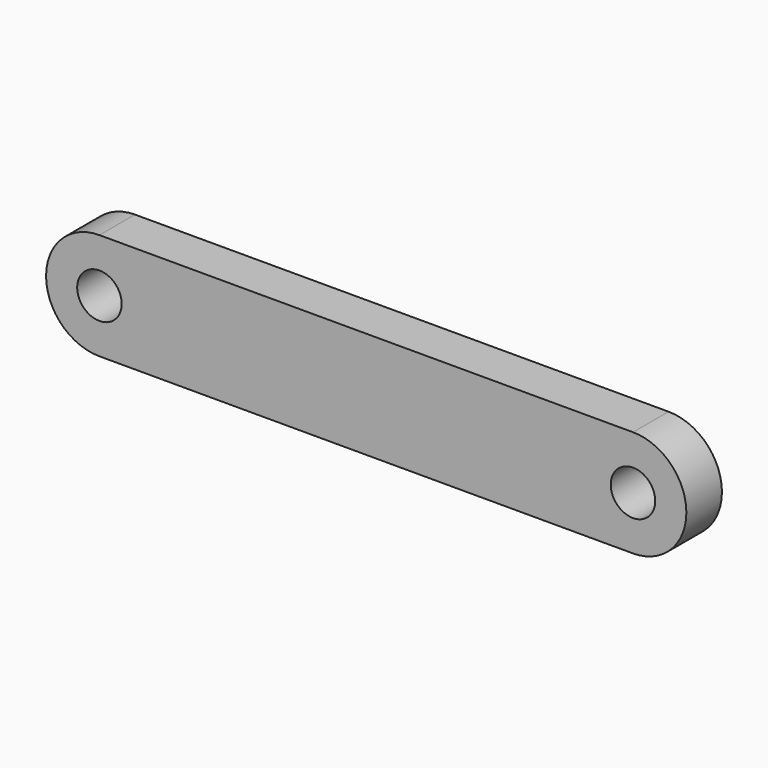
from build123d import *

# Parameters (mm, degrees)
F0_R     = 2.5
F1_DEPTH = 5


# Not quite as in the source:
# - a feature names something its author has since deleted; it is built from what else it names


with BuildPart() as f1:
    # F0 (on Front) → F1 (new body)
    with BuildSketch(Plane.XZ):
        with BuildLine():
            ThreePointArc((0, 12), (-6, 6), (0, 0))
            Line((0, 0), (60, 0))
            ThreePointArc((60, 0), (66, 6), (60, 12))
            Line((60, 12), (0, 12))
        make_face()
        with Locations((0, 6)):
            Circle(F0_R, mode=Mode.SUBTRACT)
        with Locations((60, 6)):
            Circle(F0_R, mode=Mode.SUBTRACT)
    extrude(amount=F1_DEPTH)


solid = f1.part
